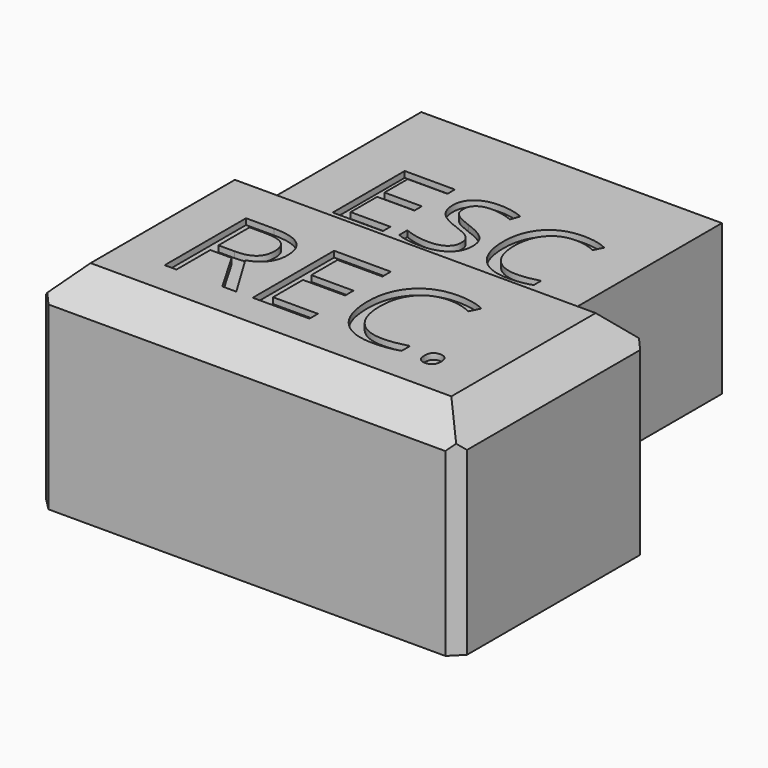
from build123d import *

# Parameters (mm, degrees)
F0_W         = 70
F0_H         = 40
F1_DEPTH     = 35
F2_SIZE      = 5
F3_SIZE      = 2
F4_W         = 50
F4_H         = 40
F5_DEPTH     = 25
F6_TEXT_SIZE = 20.9635382311
F7_DEPTH     = 1
F8_TEXT_SIZE = 23.6979142452
F9_DEPTH     = 1


# Not quite as in the source:
# - Text() gives the source's letters only with a copy of the font that has no kerning and outlines rounded to 1/6400 em; it was checked with that copy


with BuildPart() as f1:
    # F0 (on Top) → F1 (new body)
    with BuildSketch(Plane.XY):
        with Locations((35, 20)):
            Rectangle(F0_W, F0_H)
    extrude(amount=F1_DEPTH)

    # F2
    f2_edges = [f1.edges().sort_by_distance(p)[0] for p in [
        (0, 20, 35),
        (35, 0, 35),
        (70, 20, 35),
        (35, 40, 35),
    ]]
    chamfer(f2_edges, length=F2_SIZE)

    # F3
    f3_edges = [f1.edges().sort_by_distance(p)[0] for p in [
        (0, 40, 15),
        (0, 0, 15),
        (70, 0, 15),
        (70, 40, 15),
    ]]
    chamfer(f3_edges, length=F3_SIZE)

    # F4 (on face) → F5 (join)
    with BuildSketch(Plane(origin=(0, 0, 0), x_dir=(1, 0, 0), z_dir=(0, 0, -1))):
        with Locations((25, -60)):
            Rectangle(F4_W, F4_H)
    extrude(amount=-F5_DEPTH)

    # F6 (on face) → F7 (cut)
    with BuildSketch(Plane.XY.offset(25)):
        with Locations((6.617187988, 50.7460944355)):
            Text('ESC', F6_TEXT_SIZE, font='Open Sans', text_align=(TextAlign.LEFT, TextAlign.BOTTOM))
    extrude(amount=-F7_DEPTH, mode=Mode.SUBTRACT)

    # F8 (on face) → F9 (cut)
    with BuildSketch(Plane.XY.offset(35)):
        with Locations((10.5546889827, 10.5507820845)):
            Text('REC.', F8_TEXT_SIZE, font='Open Sans', text_align=(TextAlign.LEFT, TextAlign.BOTTOM))
    extrude(amount=-F9_DEPTH, mode=Mode.SUBTRACT)


solid = f1.part
